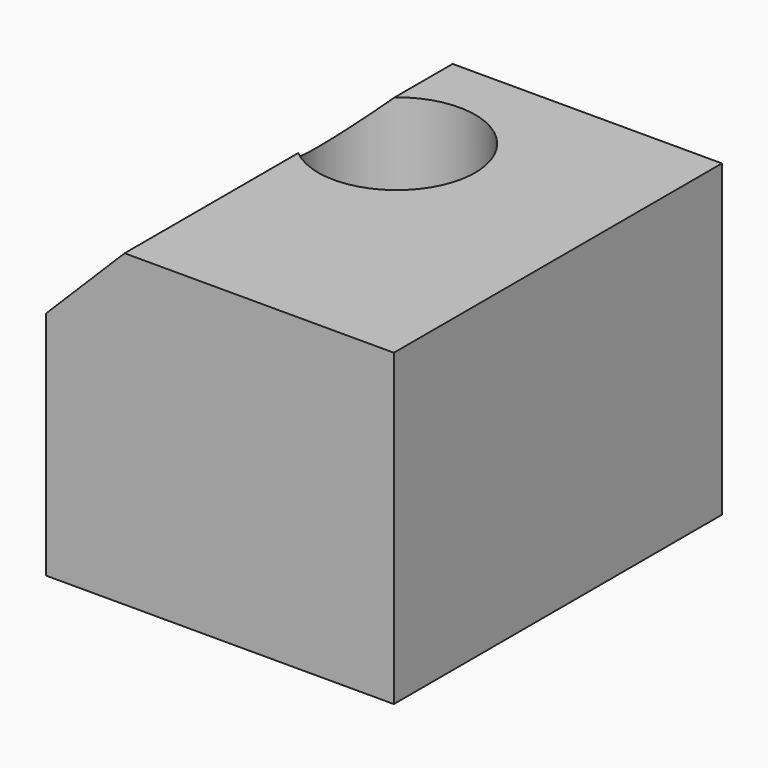
from build123d import *

# Parameters (mm, degrees)
F0_W        = 112.5368224457
F0_H        = 100.0910364091
F1_DEPTH    = 132.68445
F3_D        = 50.8
F4_T1_DEPTH = 263.3259457887


# Not quite as in the source:
# - a fillet or chamfer that OpenCascade refuses, or shapes differently, is made with other operations: its cross-section is extruded or revolved along the edge and cut away or added


with BuildPart() as f1:
    # F0 (on Front) → F1 (new body)
    with BuildSketch(Plane.XZ):
        with Locations((-44.0393215977, 6.0430746526)):
            Rectangle(F0_W, F0_H)
    extrude(amount=F1_DEPTH)

    # F3 (through all)
    with Locations(Plane(origin=(0, 0, -44.002443552), x_dir=(1, 0, 0), z_dir=(0, 0, -1))):
        with Locations((-58.6555227637, 42.9257005453)):
            Hole(F3_D / 2)

    # F4: chamfer of 25.4 on 1 edges, made by hand

    # F4_s2 → F4_t1 (cut)
    with BuildSketch(Plane.XZ.offset(-65.3207478943)):
        Polygon((-74.9077328205, 56.0885928571), (-100.3077328205, 30.6885928571), (-100.3077328205, 56.0885928571), align=None)
    extrude(amount=F4_T1_DEPTH, mode=Mode.SUBTRACT)


solid = f1.part
